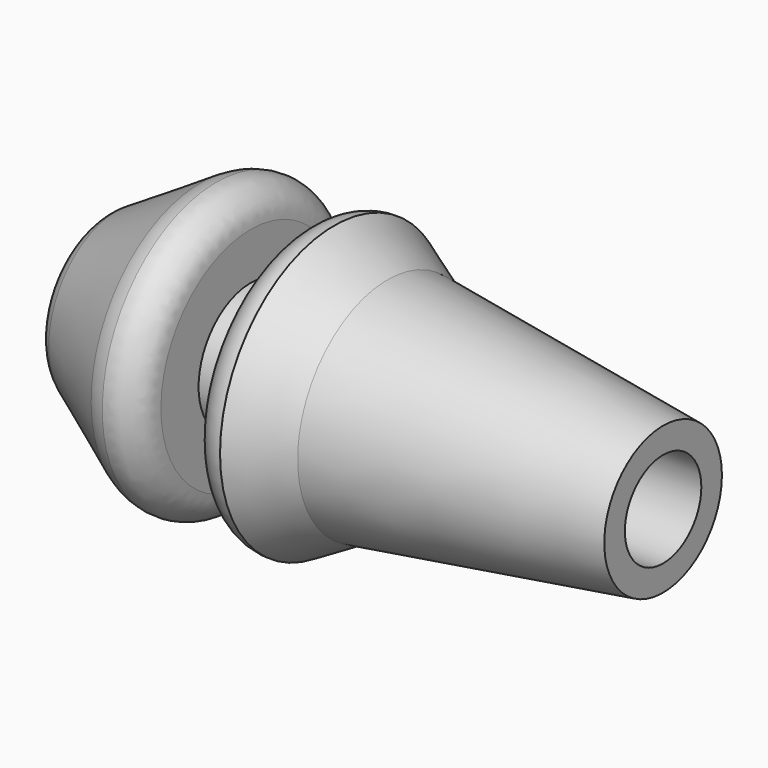
from build123d import *

# Parameters (mm, degrees)
F2_F1_R  = 6.35
F2_F2_R  = 6.35
F3_R     = 7.9375
F4_DEPTH = 93.7661007047
F6_R     = 5.08


# Not quite as in the source:
# - two fillets or chamfers of one size are made in one step


with BuildPart() as f1:
    # F0 (on Top) → F1 (revolve)
    with BuildSketch(Plane.XY):
        Polygon((-39.1627885401, 12.2120529413), (-39.1627885401, 0), (54.6033121645, 0), (54.6033121645, 12.2120529413), (8.8432114571, 18.6689998955), (0, 23.7222649157), (-5.1936330274, 23.7222649157), (-5.1936330274, 10.8083682135), (-13.8964727521, 10.8083682135), (-13.8964727521, 23.7222649157), (-20.6341594458, 23.7222649157), align=None)
    revolve(axis=Axis((7.7202618122, 0, 0), (1, 0, 0)))

    # F2: fillet of radius 6.35 on 2 edges, made by hand

    # F2_f1
    f2_f1_edges = [f1.edges().sort_by_distance(p)[0] for p in [
        (-39.1627885401, -12.2120529413, 0),
    ]]
    fillet(f2_f1_edges, radius=F2_F1_R)

    # F2_f2
    f2_f2_edges = [f1.edges().sort_by_distance(p)[0] for p in [
        (-20.6341594458, -23.7222649157, 0),
    ]]
    fillet(f2_f2_edges, radius=F2_F2_R)

    # F3 (on face) → F4 (cut, through all)
    with BuildSketch(Plane.YZ.offset(54.6033121645)):
        Circle(F3_R)
    extrude(amount=-F4_DEPTH, mode=Mode.SUBTRACT)

    # F6
    f6_edges = [f1.edges().sort_by_distance(p)[0] for p in [
        (-13.896473, -23.722265, 0),
        (-5.193633, -23.722265, 0),
    ]]
    fillet(f6_edges, radius=F6_R)


solid = f1.part
